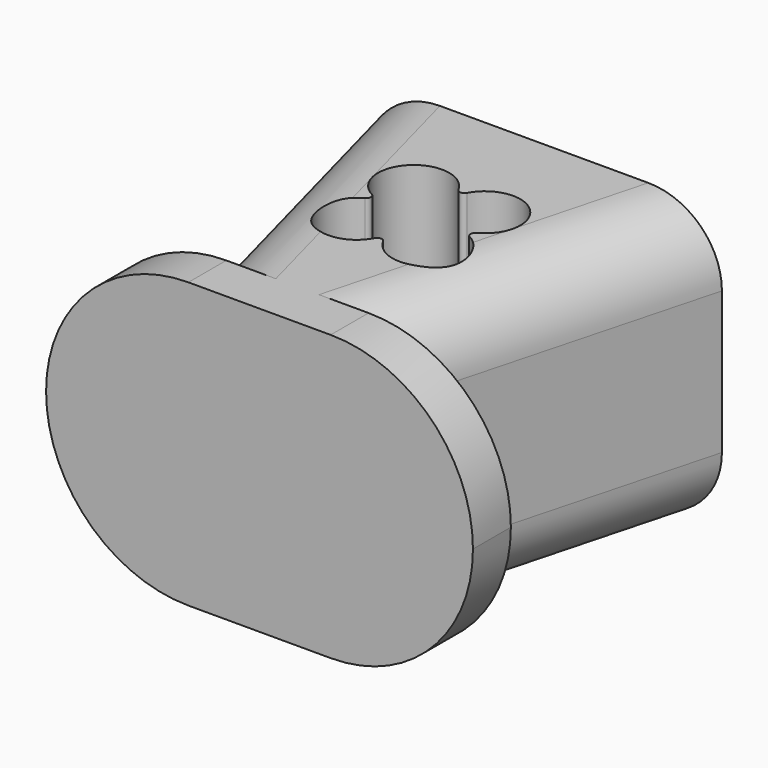
from build123d import *

# Parameters (mm, degrees)
F1_DEPTH    = 6
F2_F1_R     = 0.2
F2_F2_R     = 0.2
F3_T4_DEPTH = 28.4585903453
F3_T9_DEPTH = 28.4585903453
F4_R        = 5.99999


# Not quite as in the source:
# - a fillet or chamfer that OpenCascade refuses, or shapes differently, is made with other operations: its cross-section is extruded or revolved along the edge and cut away or added
# - a fillet or chamfer is up to 0.001 mm smaller than in the source, because OpenCascade refuses the exact size


with BuildPart() as f1:
    # F0 (on Top) → F1 (new body)
    with BuildSketch(Plane.XY):
        Polygon((-7.5, 8), (-4.418584287, -3.5), (4.418584287, -3.5), (7.5, 8), align=None)
        with BuildLine():
            ThreePointArc((-1.5, 1.5), (-2.5606601718, 4.0606601718), (0, 3))
            ThreePointArc((0, 3), (2.5606601718, 4.0606601718), (1.5, 1.5))
            ThreePointArc((1.5, 1.5), (2.5606601718, -1.0606601718), (0, 0))
            ThreePointArc((0, 0), (-2.5606601718, -1.0606601718), (-1.5, 1.5))
        make_face(mode=Mode.SUBTRACT)
        Polygon((-9, -5), (-9, -7), (9, -7), (9, -5), (4.0166604984, -5), (-4.0166604984, -5), align=None)
        Polygon((-4.418584287, -3.5), (-4.0166604984, -5), (4.0166604984, -5), (4.418584287, -3.5), align=None)
    extrude(amount=F1_DEPTH)

    # F2: fillet of radius 0.2 on 4 edges, made by hand

    # F2_f1
    f2_f1_edges = [f1.edges().sort_by_distance(p)[0] for p in [
        (-1.5, 1.5, 3),
        (0, 3, 3),
        (1.5, 1.5, 3),
    ]]
    fillet(f2_f1_edges, radius=F2_F1_R)

    # F2_f2
    f2_f2_edges = [f1.edges().sort_by_distance(p)[0] for p in [
        (0, 0, 3),
    ]]
    fillet(f2_f2_edges, radius=F2_F2_R)

    # F3: fillet of radius 3 on 2 edges, made by hand


with BuildPart() as f3_tool2:
    # F3_s3 → F3_t4 (new body)
    with BuildSketch(Plane(origin=(-4.4435475741, 16.5835453123, 0), x_dir=(0, 0, 1), z_dir=(0.2588190451, -0.9659258263, 0))):
        with BuildLine():
            ThreePointArc((3, 5.1738913363), (5.1213203436, 4.2952116799), (6, 2.1738913363))
            Line((6, 2.1738913363), (6, 5.1738913363))
            Line((6, 5.1738913363), (3, 5.1738913363))
        make_face()
    extrude(amount=F3_T4_DEPTH)

    split(bisect_by=Plane.XZ.offset(5), keep=Keep.BOTTOM)


with BuildPart() as f1_1:
    add(f1.part)

    # F3_t1: cut F3_tool2
    add(f3_tool2.part, mode=Mode.SUBTRACT)


with BuildPart() as f3_tool7:
    # F3_s8 → F3_t9 (new body)
    with BuildSketch(Plane(origin=(-2.9220776041, -10.905342082, 0), x_dir=(0, 0, 1), z_dir=(0.2588190451, 0.9659258263, 0))):
        with BuildLine():
            ThreePointArc((3, 5.1738913363), (5.1213203436, 4.2952116799), (6, 2.1738913363))
            Line((6, 2.1738913363), (6, 5.1738913363))
            Line((6, 5.1738913363), (3, 5.1738913363))
        make_face()
    extrude(amount=F3_T9_DEPTH)

    split(bisect_by=Plane.XZ.offset(5), keep=Keep.BOTTOM)


with BuildPart() as f1_2:
    add(f1_1.part)

    # F3_t6: cut F3_tool7
    add(f3_tool7.part, mode=Mode.SUBTRACT)

    # F4 (radius 6 in the source; OpenCascade refuses exactly that, so slightly less here)
    f4_edges = [f1_2.edges().sort_by_distance(p)[0] for p in [
        (9, -6, 6),
        (-9, -6, 6),
    ]]
    fillet(f4_edges, radius=F4_R)

    # F5: F1 across plane


with BuildPart() as f1_3:
    add(f1_2.part)
    add(f1_2.part.mirror(Plane.XY))


solid = f1_3.part
